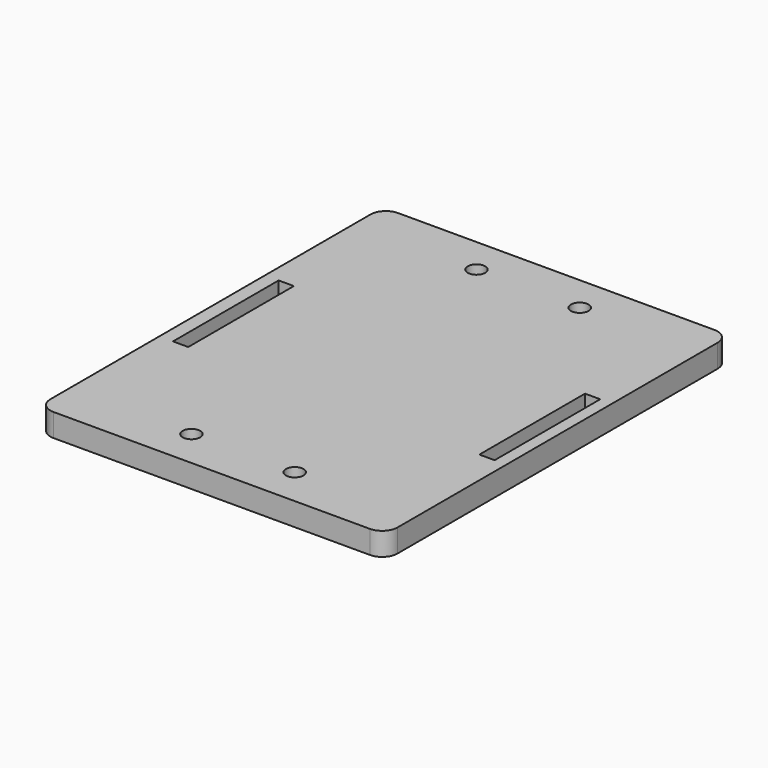
from build123d import *

# Parameters (mm, degrees)
F0_W     = 115.1548996568
F0_H     = 142.901070416
F1_DEPTH = 7.62
F2_R     = 5.08
F3_W     = 5.0534754992
F3_H     = 43.796794489
F3_R     = 2.9202239124
F4_DEPTH = 7.62


# Not quite as in the source:
# - a feature names something its author has since deleted; it is built from what else it names


with BuildPart() as f1:
    # F0 (on Top) → F1 (new body)
    with BuildSketch(Plane.XY):
        with Locations((-0.3047175705, -0.2807490528)):
            Rectangle(F0_W, F0_H)
    extrude(amount=F1_DEPTH)

    # F2
    f2_edges = [f1.edges().sort_by_distance(p)[0] for p in [
        (-57.882167, -71.731284, 3.81),
        (-57.882167, 71.169786, 3.81),
        (57.272732, -71.731284, 3.81),
        (57.272732, 71.169786, 3.81),
    ]]
    fillet(f2_edges, radius=F2_R)

    # F3 (on face) + F0 (on Top) → F4 (cut)
    with BuildSketch(Plane.XY.offset(7.62)):
        with Locations((-50.8155077696, 0.4211226478)):
            Rectangle(F3_W, F3_H)
        with Locations((17.1256698668, 59.0975955129)):
            Circle(F3_R)
        with Locations((50.8155077696, 0.4211226478)):
            Rectangle(F3_W, F3_H)
        with Locations((-17.1256698668, 59.0975955129)):
            Circle(F3_R)
        with Locations((-17.1256698668, -59.0975955129)):
            Circle(F3_R)
        with Locations((17.1256698668, -59.0975955129)):
            Circle(F3_R)
    with BuildSketch(Plane.XY):
        with Locations((-0.3047175705, -0.2807490528)):
            Rectangle(F0_W, F0_H)
    extrude(amount=-F4_DEPTH, mode=Mode.SUBTRACT)


solid = f1.part
